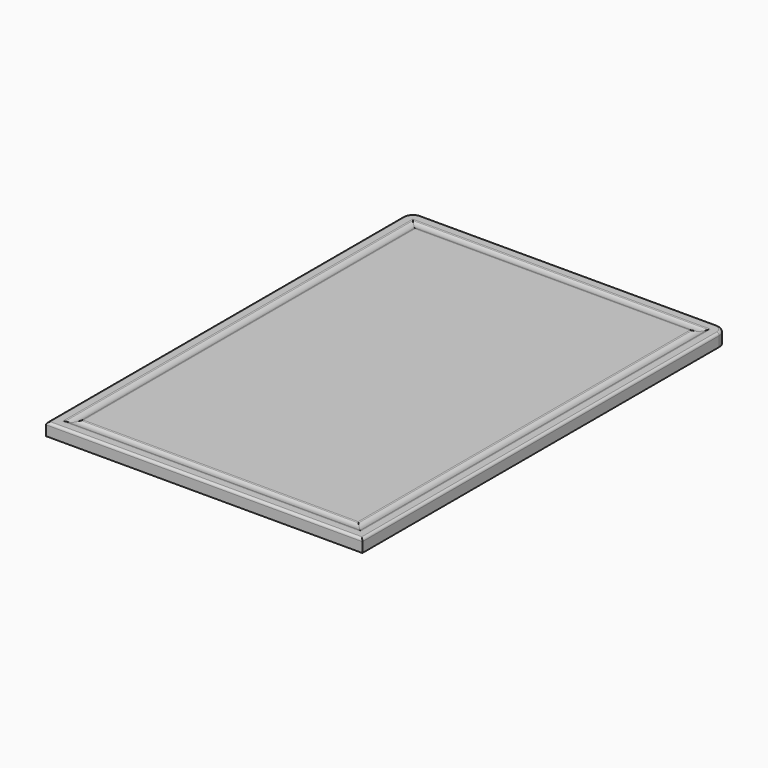
from build123d import *

# Parameters (mm, degrees)
F0_W        = 632.46
F0_H        = 911.86
F1_DEPTH    = 25
F3_R        = 18.1666666667
F6_T1_DEPTH = 124.9995000013
F7_R        = 5


# Not quite as in the source:
# - a fillet or chamfer that OpenCascade refuses, or shapes differently, is made with other operations: its cross-section is extruded or revolved along the edge and cut away or added


with BuildPart() as f1:
    # F0 (on Top) → F1 (new body)
    with BuildSketch(Plane.XY):
        Rectangle(F0_W, F0_H)
    extrude(amount=-F1_DEPTH)


with BuildPart() as f4:
    # F4: sweep along a path in F2
    with BuildLine(Plane.XY) as f4_path:
        Line((-286.2199, 425.9199), (286.2199, 425.9199))
        Line((286.2199, 425.9199), (286.2199, -425.9199))
        Line((286.2199, -425.9199), (-286.2199, -425.9199))
        Line((-286.2199, -425.9199), (-286.2199, 425.9199))
    # F3 (on Front) → F4 (sweep)
    with BuildSketch(Plane.XZ):
        with Locations((286.2199, 15.1666666667)):
            Circle(F3_R)
    sweep(path=f4_path.line, transition=Transition.RIGHT)


with BuildPart() as f1_1:
    add(f1.part)

    # F5: cut F4
    add(f4.part, mode=Mode.SUBTRACT)

    # F6: fillet of radius 20 on 2 edges, made by hand

    # F6_s2 → F6_t1 (cut)
    with BuildSketch(Plane.XY.offset(-74.9997500006)):
        with BuildLine():
            ThreePointArc((296.2301, 455.9301), (310.3722356237, 450.0722356237), (316.2301, 435.9301))
            Line((316.2301, 435.9301), (316.6301, 435.9301))
            ThreePointArc((316.6301, 435.9301), (316.63, 445.93005), (316.63, 455.93))
            Line((316.63, 455.93), (316.23, 456.33))
            ThreePointArc((316.23, 456.33), (306.23005, 456.33), (296.2301, 456.3301))
            Line((296.2301, 456.3301), (296.2301, 455.9301))
        make_face()
        with BuildLine():
            ThreePointArc((-296.2301, 455.9301), (-310.3722356237, 450.0722356237), (-316.2301, 435.9301))
            Line((-316.2301, 435.9301), (-316.6301, 435.9301))
            ThreePointArc((-316.6301, 435.9301), (-316.63, 445.93005), (-316.63, 455.93))
            Line((-316.63, 455.93), (-316.23, 456.33))
            ThreePointArc((-316.23, 456.33), (-306.23005, 456.33), (-296.2301, 456.3301))
            Line((-296.2301, 456.3301), (-296.2301, 455.9301))
        make_face()
    extrude(amount=F6_T1_DEPTH, mode=Mode.SUBTRACT)

    # F7
    f7_edges = [f1_1.edges().sort_by_distance(p)[0] for p in [
        (0, 415.9199, 0),
        (276.2199, 0, 0),
        (0, -415.9199, 0),
        (-276.2199, 0, 0),
        (0, 455.93, 0),
        (-310.372236, 450.072236, 0),
        (-316.23, -9.968327, 0),
        (310.372236, 450.072236, 0),
        (316.23, -9.968327, 0),
        (0, -455.93, 0),
        (-296.2199, 0, 0),
        (0, -435.9199, 0),
        (0, 435.9199, 0),
        (296.2199, 0, 0),
    ]]
    fillet(f7_edges, radius=F7_R)


solid = f1_1.part
